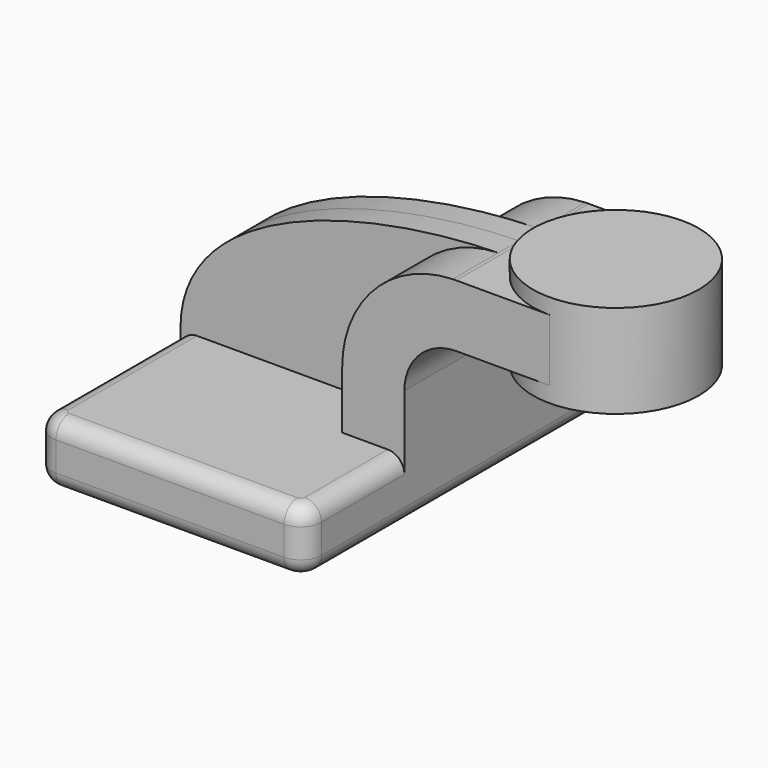
from build123d import *

# Parameters (mm, degrees)
F1_DEPTH     = 63.5
F0_W         = 25.4
F0_H         = 19.05
F2_DEPTH     = 25.4
F3_DEPTH     = 7.9375
F5_R         = 6.35
F6_R         = 5.08
F7_T1_DEPTH  = 69.85
F7_T3_DEPTH  = 49.2125
F7_T5_DEPTH  = 31.75
F7_T8_ANGLE  = 90
F7_T10_ANGLE = 90
F8_R         = 5.08


# Not quite as in the source:
# - a fillet or chamfer that OpenCascade refuses, or shapes differently, is made with other operations: its cross-section is extruded or revolved along the edge and cut away or added


with BuildPart() as f1:
    # F0 (on Front) → F1 (new body, symmetric)
    with BuildSketch(Plane.XZ):
        Polygon((22.225, 9.525), (-41.275, 9.525), (-41.275, -9.525), (41.275, -9.525), (41.275, 9.525), align=None)
    extrude(amount=F1_DEPTH, both=True)

    # F0 (on Front) → F2 (join, symmetric)
    with BuildSketch(Plane.XZ):
        with BuildLine():
            Line((22.225, 27.0002), (22.225, 9.525))
            Line((22.225, 9.525), (41.275, 9.525))
            Line((41.275, 9.525), (41.275, 27.0002))
            ThreePointArc((41.275, 27.0002), (45.9246798487, 38.2255201513), (57.15, 42.8752))
            Line((57.15, 42.8752), (60.325, 42.8752))
            Line((60.325, 42.8752), (60.325, 61.9252))
            Line((60.325, 61.9252), (57.15, 61.9252))
            add(Edge.make_bspline(
                [(56.0885572702, 61.9090665575), (56.4433633619, 61.9154910812), (56.7971916203, 61.9208676872), (57.15, 61.9252)],
                knots=[110.5707934898, 110.5707934898, 110.5707934898, 110.5707934898, 111.5045361635, 111.5045361635, 111.5045361635, 111.5045361635], degree=3))
            ThreePointArc((56.0885572702, 61.9090665575), (32.0818278255, 51.3177321287), (22.225, 27.0002))
        make_face()
        with Locations((73.025, 52.4002)):
            Rectangle(F0_W, F0_H)
    extrude(amount=F2_DEPTH, both=True)

    # F0 (on Front) → F3 (join, symmetric)
    with BuildSketch(Plane.XZ):
        with BuildLine():
            add(Edge.make_bspline(
                [(-41.275, 9.525), (-41.6531258736, 45.6930648181), (14.073565129, 61.1482951996), (56.0885572702, 61.9090665575)],
                knots=[0, 0, 0, 0, 110.5707934898, 110.5707934898, 110.5707934898, 110.5707934898], degree=3))
            Line((-41.275, 9.525), (22.225, 9.525))
            Line((22.225, 9.525), (22.225, 27.0002))
            ThreePointArc((22.225, 27.0002), (32.0818278255, 51.3177321287), (56.0885572702, 61.9090665575))
        make_face()
    extrude(amount=F3_DEPTH, both=True)

    # F0 (on Front) → F4 (revolve)
    with BuildSketch(Plane.XZ):
        Polygon((85.725, 66.675), (85.725, 61.9252), (85.725, 42.8752), (85.725, 38.1), (111.125, 38.1), (111.125, 66.675), align=None)
    revolve(axis=Axis((85.725, 0, 52.3875), (0, 0, 1)))

    # F5
    f5_edges = [f1.edges().sort_by_distance(p)[0] for p in [
        (-41.275, -63.5, 0),
        (41.275, -63.5, 0),
        (41.275, 63.5, 0),
        (-41.275, 63.5, 0),
    ]]
    fillet(f5_edges, radius=F5_R)

    # F6
    f6_edges = [f1.edges().sort_by_distance(p)[0] for p in [
        (0, -63.5, -9.525),
    ]]
    fillet(f6_edges, radius=F6_R)

    # F7: fillet of radius 5.08 on 1 edges, made by hand

    # F7_s2 → F7_t1 (cut)
    with BuildSketch(Plane.YZ.offset(-34.925)):
        with BuildLine():
            ThreePointArc((58.42, 9.525), (62.0121024484, 8.0371024484), (63.5, 4.445))
            Line((63.5, 4.445), (63.5, 9.525))
            Line((63.5, 9.525), (58.42, 9.525))
        make_face()
    extrude(amount=F7_T1_DEPTH, mode=Mode.SUBTRACT)

    # F7_s4 → F7_t3 (cut)
    with BuildSketch(Plane.XZ.offset(-57.15)):
        with BuildLine():
            ThreePointArc((-36.195, 9.525), (-39.7871024484, 8.0371024484), (-41.275, 4.445))
            Line((-41.275, 4.445), (-41.275, 9.525))
            Line((-41.275, 9.525), (-36.195, 9.525))
        make_face()
    extrude(amount=F7_T3_DEPTH, mode=Mode.SUBTRACT)

    # F7_s6 → F7_t5 (cut)
    with BuildSketch(Plane.XZ.offset(-57.15)):
        with BuildLine():
            ThreePointArc((41.275, 4.445), (39.7871024484, 8.0371024484), (36.195, 9.525))
            Line((36.195, 9.525), (41.275, 9.525))
            Line((41.275, 9.525), (41.275, 4.445))
        make_face()
    extrude(amount=F7_T5_DEPTH, mode=Mode.SUBTRACT)

    # F7_s7 → F7_t8 (revolve, cut)
    with BuildSketch(Plane.XZ.offset(-57.15)):
        with BuildLine():
            ThreePointArc((41.275, 4.445), (39.7871024484, 8.0371024484), (36.195, 9.525))
            Line((36.195, 9.525), (41.275, 9.525))
            Line((41.275, 9.525), (41.275, 4.445))
        make_face()
    revolve(axis=Axis((34.925, 57.15, 9.525), (0, 0, 1)), revolution_arc=F7_T8_ANGLE, mode=Mode.SUBTRACT)

    # F7_s9 → F7_t10 (revolve, cut)
    with BuildSketch(Plane.XZ.offset(-57.15)):
        with BuildLine():
            ThreePointArc((-36.195, 9.525), (-39.7871024484, 8.0371024484), (-41.275, 4.445))
            Line((-41.275, 4.445), (-41.275, 9.525))
            Line((-41.275, 9.525), (-36.195, 9.525))
        make_face()
    revolve(axis=Axis((-34.925, 57.15, 9.525), (0, 0, -1)), revolution_arc=F7_T10_ANGLE, mode=Mode.SUBTRACT)

    # F8
    f8_edges = [f1.edges().sort_by_distance(p)[0] for p in [
        (0, -63.5, 9.525),
        (41.275, -41.275, 9.525),
        (39.415128, -61.640128, 9.525),
        (-39.415128, -61.640128, 9.525),
        (-41.275, -32.54375, 9.525),
    ]]
    fillet(f8_edges, radius=F8_R)


solid = f1.part
